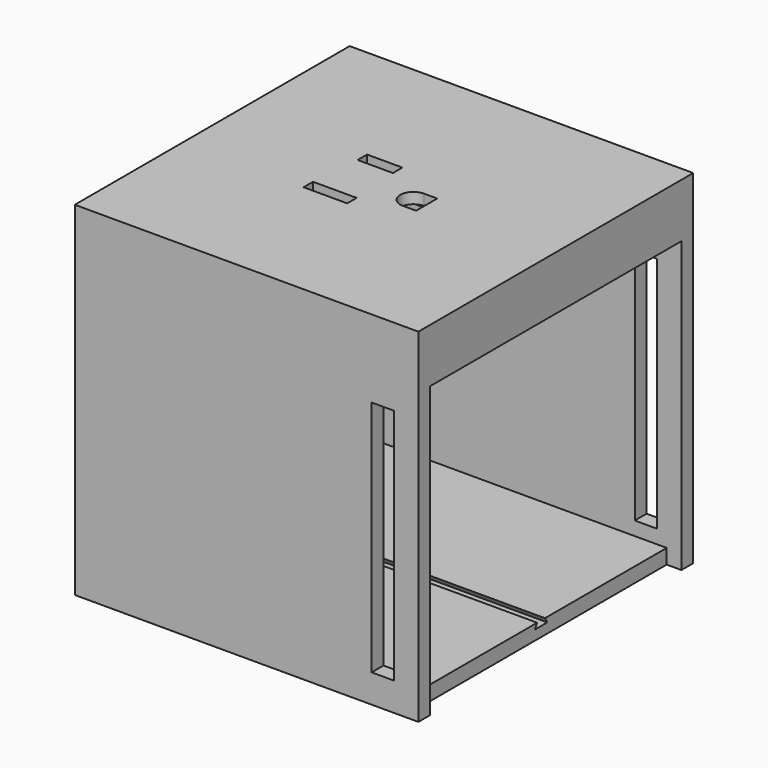
from build123d import *

# Parameters (mm, degrees)
F0_W      = 70
F0_H      = 70
F1_DEPTH  = 70
F2_T      = -3
F3_W      = 8.89
F3_H      = 2.41
F3_W_2    = 7.2
F4_DEPTH  = 2.54
F5_W      = 3
F5_H      = 64
F6_DEPTH  = 8
F7_R      = 2.05
F8_DEPTH  = 3.302
F9_W      = 4.5
F9_H      = 48.4
F10_DEPTH = 99.568
F11_W     = 67
F11_H     = 2
F12_DEPTH = 1
F12_TAPER = -30
F14_DEPTH = 0.8
F16_DEPTH = 0.8
F17_W     = 7.2
F17_H     = 1.2938163138
F17_H_2   = 4.2561836862
F17_H_3   = 6.35
F18_DEPTH = 0.8
F20_DEPTH = 0.8
F21_W     = 3
F21_H     = 64
F22_DEPTH = 4.6


# Not quite as in the source:
# - a feature names something its author has since deleted; it is built from what else it names


with BuildPart() as f1:
    # F0 (on Top) → F1 (new body)
    with BuildSketch(Plane.XY):
        with Locations((1.2258447155, 1.6609302163)):
            Rectangle(F0_W, F0_H)
    extrude(amount=F1_DEPTH)

    # F2
    f2_openings = [f1.faces().sort_by_distance(p)[0] for p in [
        (36.225845, 1.66093, 35),
    ]]
    offset(amount=F2_T, openings=f2_openings)

    # F3 (on face) → F4 (cut)
    with BuildSketch(Plane.XY.offset(70)):
        with Locations((-4.6741552845, -4.6890697837)):
            Rectangle(F3_W, F3_H)
        with BuildLine():
            ThreePointArc((7.2258447155, -1.0290697837), (9.1279619569, -0.2411870251), (9.9158447155, 1.6609302163))
            ThreePointArc((9.9158447155, 1.6609302163), (9.1279619569, 3.5630474577), (7.2258447155, 4.3509302163))
            ThreePointArc((7.2258447155, 4.3509302163), (4.5358447155, 1.6609302163), (7.2258447155, -1.0290697837))
        make_face()
        with BuildLine():
            Line((9.9158447155, -1.0290697837), (9.9158447155, 1.6609302163))
            ThreePointArc((9.9158447155, 1.6609302163), (9.1279619569, -0.2411870251), (7.2258447155, -1.0290697837))
            Line((7.2258447155, -1.0290697837), (9.9158447155, -1.0290697837))
        make_face()
        with Locations((-4.6741552845, 8.0109302163)):
            Rectangle(F3_W_2, F3_H)
        with BuildLine():
            ThreePointArc((7.2258447155, 4.3509302163), (9.1279619569, 3.5630474577), (9.9158447155, 1.6609302163))
            Line((9.9158447155, 1.6609302163), (9.9158447155, 4.3509302163))
            Line((9.9158447155, 4.3509302163), (7.2258447155, 4.3509302163))
        make_face()
    extrude(amount=-F4_DEPTH, mode=Mode.SUBTRACT)

    # F5 (on face) → F6 (join)
    with BuildSketch(Plane(origin=(0, 0, 67), x_dir=(1, 0, 0), z_dir=(0, 0, -1))):
        with Locations((34.7258447155, -1.6609302163)):
            Rectangle(F5_W, F5_H)
    extrude(amount=F6_DEPTH)

    # F7 (on face) → F8 (cut)
    with BuildSketch(Plane(origin=(-33.7741552845, 0, 0), x_dir=(0, -1, 0), z_dir=(-1, 0, 0))):
        with Locations((-1.6609302163, 25.8598876931)):
            Circle(F7_R)
    extrude(amount=-F8_DEPTH, mode=Mode.SUBTRACT)

    # F9 (on face) → F10 (cut)
    with BuildSketch(Plane.XZ.offset(33.3390697837)):
        with Locations((28.9758447155, 30)):
            Rectangle(F9_W, F9_H)
    extrude(amount=-F10_DEPTH, mode=Mode.SUBTRACT)

    # F11 (on face) → F12 (cut)
    with BuildSketch(Plane.XY.offset(3)):
        with Locations((2.7258447155, 1.6609302163)):
            Rectangle(F11_W, F11_H)
    extrude(amount=-F12_DEPTH, taper=F12_TAPER, mode=Mode.SUBTRACT)

    # F13 (on face) → F14 (cut)
    with BuildSketch(Plane(origin=(0, 0, 67), x_dir=(1, 0, 0), z_dir=(0, 0, -1))):
        Polygon((-30.7741552845, -0.0109302163), (-30.7741552845, -3.3109302163), (1.0258447155, -3.3109302163), (1.7764000655, -4.6109302163), (1.7764000655, -5.1109302163), (12.5788900655, -5.1109302163), (12.5788900655, -4.6109302163), (13.3294454154, -3.3109302163), (33.2258447155, -3.3109302163), (33.2258447155, -0.0109302163), (13.3294454154, -0.0109302163), (12.5788900655, 1.2890697837), (12.5788900655, 1.7890697837), (1.7764000655, 1.7890697837), (1.7764000655, 1.2890697837), (1.0258447155, -0.0109302163), align=None)
    extrude(amount=-F14_DEPTH, mode=Mode.SUBTRACT)

    # F15 (on face) → F16 (cut)
    with BuildSketch(Plane(origin=(0, 0, 67), x_dir=(1, 0, 0), z_dir=(0, 0, -1))):
        Polygon((-30.7741552845, 5.0452534699), (-30.7741552845, 4.2452534699), (-12.6326995774, 4.2452534699), (-9.1191552845, 3.0155129674), (-0.2291552845, 3.0155129674), (3.2843890084, 4.2452534699), (33.2258447155, 4.2452534699), (33.2258447155, 5.0452534699), (3.2843890084, 5.0452534699), (-0.2291552845, 6.2749939724), (-9.1191552845, 6.2749939724), (-12.6326995774, 5.0452534699), align=None)
    extrude(amount=-F16_DEPTH, mode=Mode.SUBTRACT)

    # F17 (on face) → F18 (cut)
    with BuildSketch(Plane(origin=(0, 0, 67), x_dir=(1, 0, 0), z_dir=(0, 0, -1))):
        with Locations((29.6258447155, 5.6921616268)):
            Rectangle(F17_W, F17_H)
        with Locations((29.6258447155, 2.1171616268)):
            Rectangle(F17_W, F17_H_2)
        with Locations((29.6258447155, -6.4859302163)):
            Rectangle(F17_W, F17_H_3)
    extrude(amount=-F18_DEPTH, mode=Mode.SUBTRACT)

    # F19 (on face) → F20 (cut)
    with BuildSketch(Plane(origin=(0, 0, 67), x_dir=(1, 0, 0), z_dir=(0, 0, -1))):
        Polygon((26.0258447155, -8.4106897138), (26.0258447155, -7.6106897138), (2.4393890084, -7.6106897138), (-1.0741552845, -6.3809492113), (-8.2741552845, -6.3809492113), (-11.7876995774, -7.6106897138), (-30.7741552845, -7.6106897138), (-30.7741552845, -8.4106897138), (-11.7876995774, -8.4106897138), (-8.2741552845, -9.6404302163), (-1.0741552845, -9.6404302163), (2.4393890084, -8.4106897138), align=None)
    extrude(amount=-F20_DEPTH, mode=Mode.SUBTRACT)

    # F21 (on face) → F22 (cut)
    with BuildSketch(Plane(origin=(0, 0, 0), x_dir=(1, 0, 0), z_dir=(0, 0, -1))):
        with Locations((34.7258447155, -1.6609302163)):
            Rectangle(F21_W, F21_H)
    extrude(amount=-F22_DEPTH, mode=Mode.SUBTRACT)


solid = f1.part
